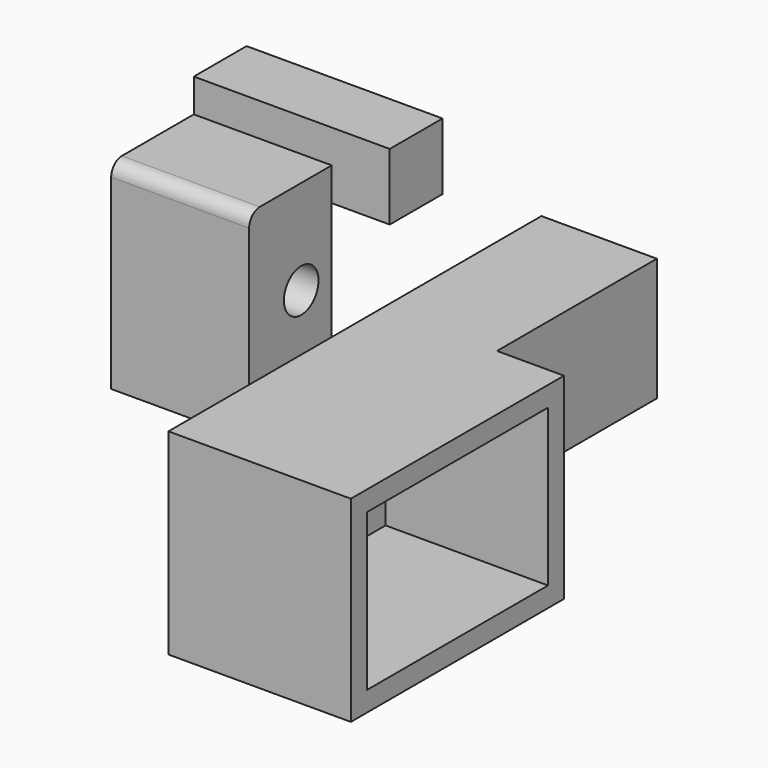
from build123d import *

# Parameters (mm, degrees)
F0_W        = 52.6178367436
F0_H        = 39.3761303276
F1_DEPTH    = 76.2
F2_R        = 5.08
F3_R        = 8.240513031
F4_DEPTH    = 52.6188367436
F6_DEPTH    = 12.7
F7_T        = 2.54
F7_T3_DEPTH = 57.6978367436
F7_T5_DEPTH = 17.78
F8_W        = 69.5647448301
F8_H        = 74.9455988407
F9_DEPTH    = 101.6
F10_T       = -7.62
F11_W       = 44.0154448152
F11_H       = 46.9202438835
F12_DEPTH   = 76.2


# Not quite as in the source:
# - a shell that OpenCascade refuses in one call is made with other operations: the cavity is built on its own and cut out


with BuildPart() as f1:
    # F0 (on Top) → F1 (new body)
    with BuildSketch(Plane.XY):
        with Locations((-69.2907851189, -5.140860565)):
            Rectangle(F0_W, F0_H)
    extrude(amount=F1_DEPTH)

    # F2
    f2_edges = [f1.edges().sort_by_distance(p)[0] for p in [
        (-69.290785, -24.828926, 76.2),
    ]]
    fillet(f2_edges, radius=F2_R)

    # F3 (on face) → F4 (cut, through all)
    with BuildSketch(Plane.YZ.offset(-42.9818667471)):
        with Locations((0, 40.1053540409)):
            Circle(F3_R)
    extrude(amount=-F4_DEPTH, mode=Mode.SUBTRACT)

    # F5 (on face) → F6 (join, symmetric)
    with BuildSketch(Plane.XY.offset(76.2)):
        Polygon((-95.5997034907, 39.7155843675), (-95.5997034907, 14.5472045988), (-42.9818667471, 14.5472045988), (-20.8651479334, 14.5472045988), (-20.8651479334, 39.7155843675), align=None)
    extrude(amount=F6_DEPTH, both=True)

    # F7: shell of thickness 2.54, made by hand


with BuildPart() as f7_core1:
    # F7_t2: copy of F1
    add(f1.part)

    # the walls: a layer under each face that stays
    f7_faces = [f7_core1.faces().sort_by_distance(p)[0] for p in [
        (-95.5997034907, 7.4433293194, 44.45),
        (-69.2907851189, -24.8289257288, 35.56),
        (-69.2907851189, -23.3410281772, 74.7121024484),
        (-69.2907851189, -5.140860565, 0),
        (-69.2907851189, -2.600860565, 76.2),
        (-69.2907851189, -8.240513031, 40.1053540409),
        (-42.9818667471, -18.2662373409, 63.5),
        (-83.1439442312, 14.5472045988, 84.6666666667),
        (-58.232425712, 27.1313944831, 63.5),
        (-58.232425712, 27.1313944831, 88.9),
        (-20.8651479334, 27.1313944831, 76.2),
    ]]
    thicken(f7_faces, amount=-F7_T, mode=Mode.SUBTRACT)

    # F7_s4 → F7_t3 (cut)
    with BuildSketch(Plane.YZ.offset(-98.1397034907)):
        Polygon((14.5218045988, 76.2254), (14.5472045988, 73.66), (17.0872045988, 73.66), (17.0872045988, 76.2), align=None)
    extrude(amount=F7_T3_DEPTH, mode=Mode.SUBTRACT)

    # F7_s6 → F7_t5 (cut)
    with BuildSketch(Plane.XY.offset(60.96)):
        Polygon((-42.9564667471, 14.5218045988), (-45.5218667471, 14.5472045988), (-45.5218667471, 17.0872045988), (-42.9818667471, 17.0872045988), align=None)
    extrude(amount=F7_T5_DEPTH, mode=Mode.SUBTRACT)


with BuildPart() as f1_1:
    add(f1.part)

    # what is left inside the walls is the cavity
    f7_cavity = [f7_core1.part.solids().sort_by_distance(p)[0] for p in [
        (-69.290785, -22.263526, 48.26),
    ]]
    add(f7_cavity, mode=Mode.SUBTRACT)


with BuildPart() as f9:
    # F8 (on Front) → F9 (new body)
    with BuildSketch(Plane.XZ):
        with Locations((22.4474929273, 6.6017955542)):
            Rectangle(F8_W, F8_H)
    extrude(amount=F9_DEPTH)

    # F10
    f10_openings = [f9.faces().sort_by_distance(p)[0] for p in [
        (57.229865, -50.8, 6.601796),
    ]]
    offset(amount=F10_T, openings=f10_openings)

    # F11 (on face) → F12 (join)
    with BuildSketch(Plane(origin=(0, 0, 0), x_dir=(-1, 0, 0), z_dir=(0, 1, 0))):
        with Locations((-9.6728429198, 20.6144730328)):
            Rectangle(F11_W, F11_H)
    extrude(amount=F12_DEPTH)


solid = Compound([f1_1.part, f9.part])
